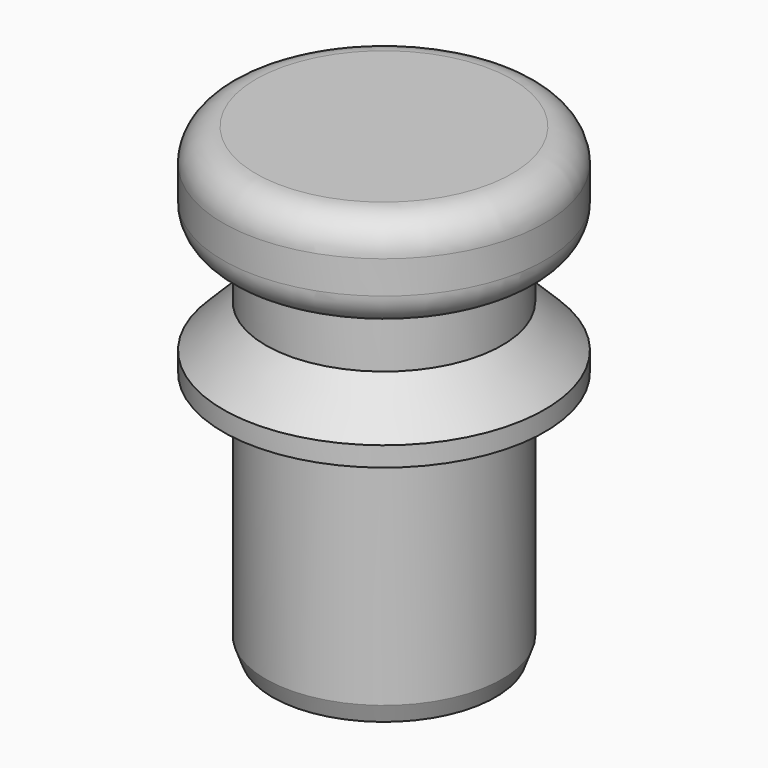
from build123d import *

# Parameters (mm, degrees)
F2_R     = 5
F3_SIZE  = 6.49999
F4_SIZE2 = 1
F4_SIZE  = 2.7474774195


# Not quite as in the source:
# - a fillet or chamfer is up to 0.001 mm smaller than in the source, because OpenCascade refuses the exact size


with BuildPart() as f1:
    # F0 (on Front) → F1 (revolve)
    with BuildSketch(Plane.XZ):
        Polygon((-18, 0), (0, 0), (0, 71), (-24.5, 71), (-24.5, 56), (-18, 56), (-18, 41), (-24.5, 41), (-24.5, 38), (-18, 38), align=None)
    revolve(axis=Axis((0, 0, 35.5), (0, 0, 1)))

    # F2
    f2_edges = [f1.edges().sort_by_distance(p)[0] for p in [
        (24.5, 0, 56),
        (24.5, 0, 71),
    ]]
    fillet(f2_edges, radius=F2_R)

    # F3 (size 6.5 in the source; OpenCascade refuses exactly that, so slightly less here)
    f3_edges = [f1.edges().sort_by_distance(p)[0] for p in [
        (18, 0, 41),
    ]]
    chamfer(f3_edges, length=F3_SIZE)

    # F4
    f4_edges = [f1.edges().sort_by_distance(p)[0] for p in [
        (18, 0, 0),
    ]]
    f4_side = f1.faces().sort_by_distance((18, 0, 19))[0]
    chamfer(f4_edges, length=F4_SIZE, length2=F4_SIZE2, reference=f4_side)


solid = f1.part
